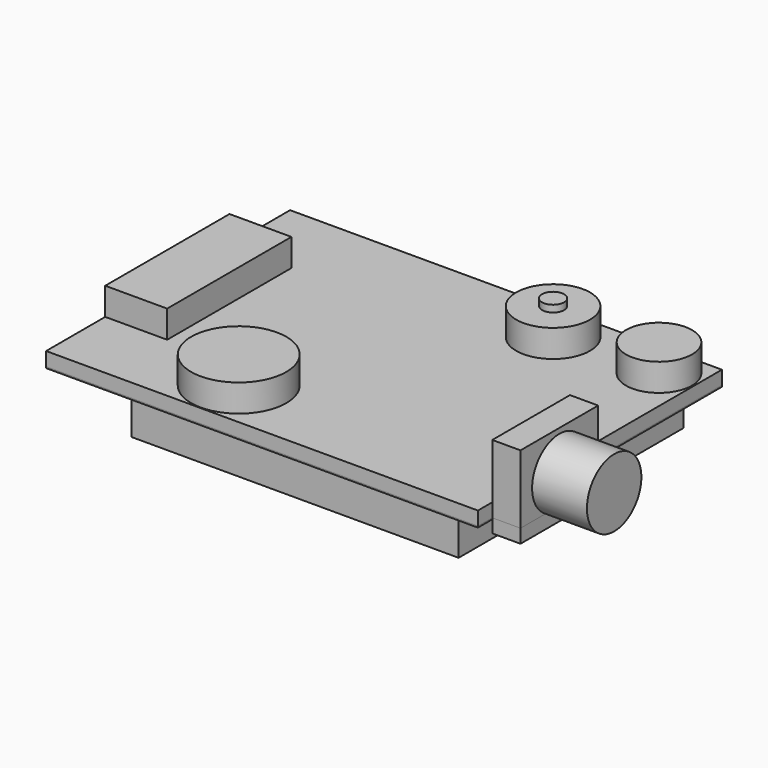
from build123d import *

# Parameters (mm, degrees)
F0_W         = 4.5180066749
F0_H         = 11.3312359899
F1_DEPTH     = 3
F0_R         = 3.4733163679
F0_R_2       = 2.6947841961
F0_R_3       = 2.4129252171
F0_W_2       = 2.0570412949
F0_H_2       = 7.0815561339
F2_DEPTH     = 1
F4_R         = 0.8035
F5_DEPTH     = 0.5
F3_R         = 2.6947841961
F3_R_2       = 2.4129252171
F3_R_3       = 3.4733163679
F6_DEPTH     = 0.1
F7_W         = 23.8446937874
F7_H         = 20.5263467506
F8_DEPTH     = 3
F9_TEXT_SIZE = 11.2482243114
F10_DEPTH    = 0.3
F11_W        = 2.0570412949
F11_H        = 7.0815561339
F12_DEPTH    = 4
F13_W        = 2.0570412949
F13_H        = 7.0815561339
F14_DEPTH    = 1
F16_DEPTH    = 4


# Not quite as in the source:
# - Text() gives the source's letters only with a copy of the font that has no kerning and outlines rounded to 1/6400 em; it was checked with that copy


with BuildPart() as f1:
    # F0 (on Top) → F1 (new body)
    with BuildSketch(Plane.XY):
        with Locations((8.9622434564, 22.6330691949)):
            Rectangle(F0_W, F0_H)
    extrude(amount=F1_DEPTH)


with BuildPart() as f1b:
    # F0 (on Top) → F1, piece 2 (new body)
    with BuildSketch(Plane.XY):
        with Locations((17.9297905415, 15.1070980355)):
            Circle(F0_R)
    extrude(amount=F1_DEPTH)


with BuildPart() as f1c:
    # F0 (on Top) → F1, piece 3 (new body)
    with BuildSketch(Plane.XY):
        with Locations((28.1899161637, 30.9482794255)):
            Circle(F0_R_2)
    extrude(amount=F1_DEPTH)

    # F4 (on face) → F5 (join)
    with BuildSketch(Plane.XY.offset(3)):
        with Locations((28.1899161637, 30.9482794255)):
            Circle(F4_R)
    extrude(amount=F5_DEPTH)


with BuildPart() as f1d:
    # F0 (on Top) → F1, piece 4 (new body)
    with BuildSketch(Plane.XY):
        with Locations((35.687699914, 31.2301516533)):
            Circle(F0_R_3)
    extrude(amount=F1_DEPTH)


with BuildPart() as f2:
    # F0 (on Top) → F2 (new body)
    with BuildSketch(Plane.XY):
        Polygon((6.7032401189, 11.5747262343), (38.2032401189, 11.5747262343), (38.2032401189, 12.8867449239), (38.2032401189, 19.9683010578), (38.2032401189, 33.8247262343), (6.7032401189, 33.8247262343), (6.7032401189, 28.2986871898), (11.2212467939, 28.2986871898), (11.2212467939, 16.9674511999), (6.7032401189, 16.9674511999), align=None)
        with Locations((17.9297905415, 15.1070980355)):
            Circle(F0_R, mode=Mode.SUBTRACT)
        with Locations((28.1899161637, 30.9482794255)):
            Circle(F0_R_2, mode=Mode.SUBTRACT)
        with Locations((35.687699914, 31.2301516533)):
            Circle(F0_R_3, mode=Mode.SUBTRACT)
        with Locations((39.2317607664, 16.4275229909)):
            Rectangle(F0_W_2, F0_H_2)
        with Locations((8.9622434564, 22.6330691949)):
            Rectangle(F0_W, F0_H)
    extrude(amount=F2_DEPTH)

    # F11 (on face) → F12 (join)
    with BuildSketch(Plane.XY.offset(1)):
        with Locations((39.2317607664, 16.4275229909)):
            Rectangle(F11_W, F11_H)
    extrude(amount=F12_DEPTH)


with BuildPart() as f6:
    # F3 (on face) → F6 (new body)
    with BuildSketch(Plane(origin=(0, 0, 0), x_dir=(1, 0, 0), z_dir=(0, 0, -1))):
        Polygon((6.7032401189, -33.8247262343), (38.2032401189, -33.8247262343), (38.2032401189, -19.9683010578), (38.2032401189, -12.8867449239), (38.2032401189, -11.5747262343), (6.7032401189, -11.5747262343), align=None)
        with Locations((28.1899161637, -30.9482794255)):
            Circle(F3_R, mode=Mode.SUBTRACT)
        with Locations((35.687699914, -31.2301516533)):
            Circle(F3_R_2, mode=Mode.SUBTRACT)
        with Locations((17.9297905415, -15.1070980355)):
            Circle(F3_R_3, mode=Mode.SUBTRACT)
        with Locations((17.9297905415, -15.1070980355)):
            Circle(F3_R_3)
        with Locations((28.1899161637, -30.9482794255)):
            Circle(F3_R)
        with Locations((35.687699914, -31.2301516533)):
            Circle(F3_R_2)
    extrude(amount=F6_DEPTH)

    # F7 (on face) → F8 (join)
    with BuildSketch(Plane(origin=(0, 0, -0.1), x_dir=(1, 0, 0), z_dir=(0, 0, -1))):
        with Locations((24.1487040184, -22.7445862256)):
            Rectangle(F7_W, F7_H)
    extrude(amount=F8_DEPTH)

    # F9 (on face) → F10 (join)
    with BuildSketch(Plane(origin=(0, 0, -3.1), x_dir=(1, 0, 0), z_dir=(0, 0, -1))):
        with Locations((14.3733192235, -26.730293408)):
            Text('VTx', F9_TEXT_SIZE, font='Open Sans', text_align=(TextAlign.LEFT, TextAlign.BOTTOM))
    extrude(amount=F10_DEPTH)


with BuildPart() as f14:
    # F13 (on face) → F14 (new body)
    with BuildSketch(Plane(origin=(0, 0, 0), x_dir=(1, 0, 0), z_dir=(0, 0, -1))):
        with Locations((39.2317607664, -16.4275229909)):
            Rectangle(F13_W, F13_H)
    extrude(amount=F14_DEPTH)


with BuildPart() as f16:
    # F15 (on face) → F16 (new body)
    with BuildSketch(Plane.YZ.offset(40.2602814138)):
        with BuildLine():
            ThreePointArc((17.6865293706, 0), (18.5829118004, 0.9074225648), (18.9105229909, 2.1401382983))
            ThreePointArc((18.9105229909, 2.1401382983), (15.1948072574, 4.2955271079), (15.1685166111, 0))
            Line((15.1685166111, 0), (17.6865293706, 0))
        make_face()
        with BuildLine():
            Line((17.6865293706, 0), (15.1685166111, 0))
            ThreePointArc((15.1685166111, 0), (16.4275229909, -0.3428617017), (17.6865293706, 0))
        make_face()
    extrude(amount=F16_DEPTH)


solid = Compound([f1.part, f1b.part, f1c.part, f1d.part, f2.part, f6.part, f14.part, f16.part])
